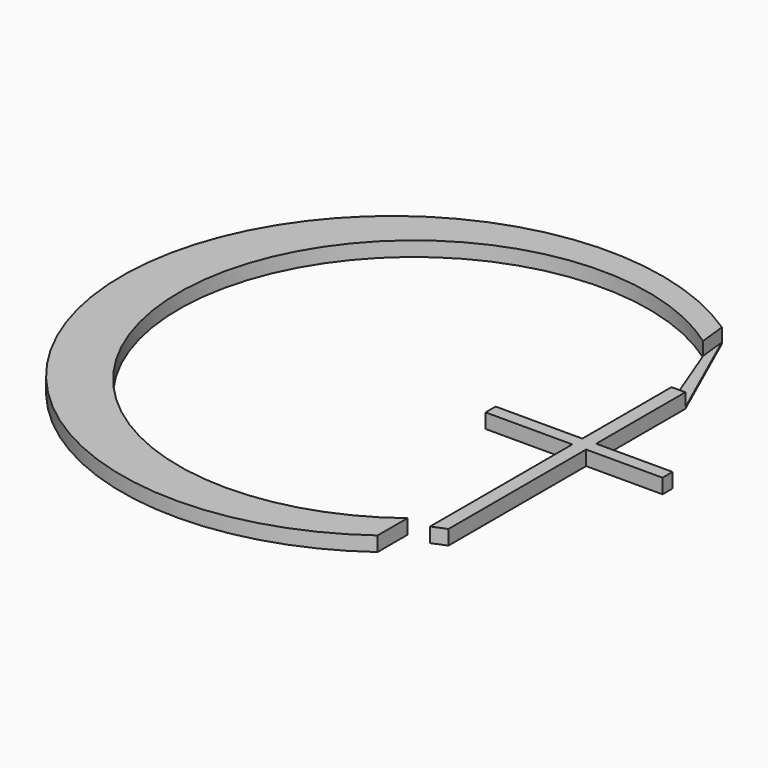
from build123d import *

# Parameters (mm, degrees)
F1_DEPTH = 2.54
F0_W     = 2.3982011194
F0_H     = 19.3259103689
F0_W_2   = 15.039473772
F0_H_2   = 2.1805369761
F0_W_3   = 13.2428539504
F2_DEPTH = 0.254


with BuildPart() as f1:
    # F0 (on Top) → F1 (new body)
    with BuildSketch(Plane.XY):
        with BuildLine():
            ThreePointArc((-11.580394581, -30.8309197426), (-77.0911936393, 0.7641380252), (-12.78355252, 34.7411856055))
            Line((-12.78355252, 34.7411856055), (-13.3079187945, 39.4789241254))
            ThreePointArc((-13.3079187945, 39.4789241254), (-86.1539650826, -0.5750175297), (-11.580394581, -37.3125635087))
            Line((-11.580394581, -37.3125635087), (-11.580394581, -30.8309197426))
        make_face()
    extrude(amount=F1_DEPTH)


with BuildPart() as f1b:
    # F0 (on Top) → F1, piece 2 (new body)
    with BuildSketch(Plane.XY):
        with Locations((-6.4710318836, 11.8434921606)):
            Rectangle(F0_W, F0_H)
        Polygon((-7.6701324433, 0), (-7.6701324433, -30.8309197426), (-5.2719313239, -29.8604014784), (-5.2719313239, 0), align=None)
        with Locations((-15.1898693293, 1.090268488)):
            Rectangle(F0_W_2, F0_H_2)
        with Locations((1.3494956513, 1.090268488)):
            Rectangle(F0_W_3, F0_H_2)
        with Locations((-6.4710318836, 1.090268488)):
            Rectangle(F0_W, F0_H_2)
    extrude(amount=F1_DEPTH)


with BuildPart() as f2:
    # F0 (on Top) → F2 (new body)
    with BuildSketch(Plane.XY):
        Polygon((-13.3079187945, 39.4789241254), (-12.78355252, 34.7411856055), (-7.6701324433, 21.506447345), (-5.2719313239, 21.506447345), align=None)
    extrude(amount=F2_DEPTH)


solid = Compound([f1.part, f1b.part, f2.part])
